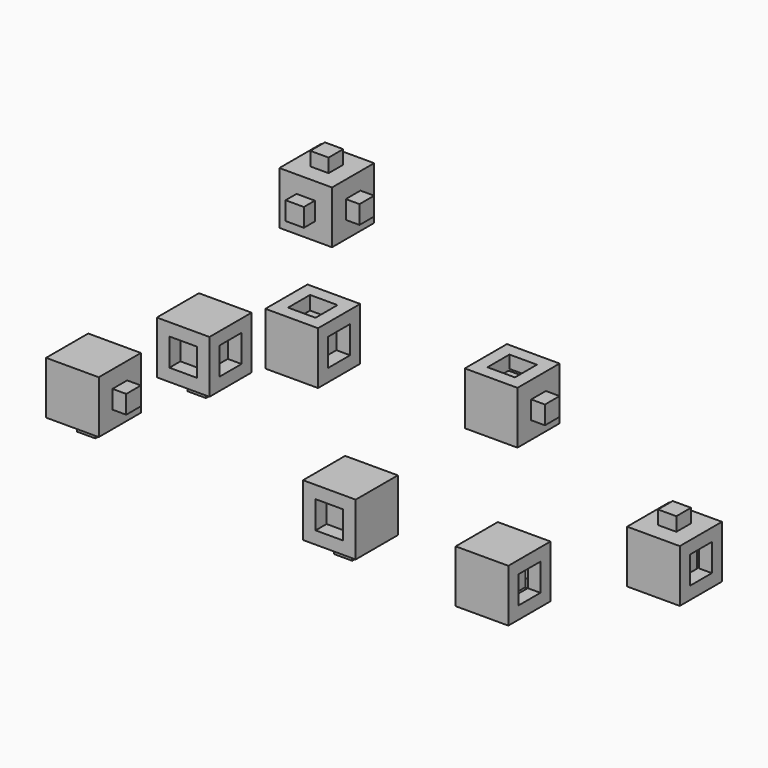
from build123d import *

# Parameters (mm, degrees)
F0_W      = 5.75
F0_H      = 5.75
F1_DEPTH  = 5.75
F2_W      = 3
F2_H      = 3
F4_DEPTH  = 1.5
F3_W      = 2
F3_H      = 2
F5_DEPTH  = 1.5
F6_W      = 3
F6_H      = 3
F7_DEPTH  = 1.5
F8_W      = 2
F8_H      = 2
F9_DEPTH  = 1.5
F10_W     = 2
F10_H     = 2
F11_DEPTH = 1.5
F12_W     = 2
F12_H     = 2
F13_DEPTH = 1.5
F14_W     = 3
F14_H     = 3
F15_DEPTH = 1.5
F16_W     = 2
F16_H     = 2
F17_DEPTH = 1.5
F18_W     = 2
F18_H     = 2
F19_DEPTH = 1.5
F20_W     = 3
F20_H     = 3
F21_DEPTH = 1.5
F22_W     = 3
F22_H     = 3
F23_DEPTH = 1.5
F24_DEPTH = 1.5
F25_W     = 2
F25_H     = 2
F26_DEPTH = 1.5
F28_W     = 2
F28_H     = 2
F29_DEPTH = 1.5
F27_W     = 2
F27_H     = 2
F30_DEPTH = 1.5
F31_W     = 2
F31_H     = 2
F32_DEPTH = 1.5
F33_W     = 3
F33_H     = 3
F34_DEPTH = 1.5
F35_W     = 3
F35_H     = 3
F36_DEPTH = 1.5
F37_W     = 2
F37_H     = 2
F38_DEPTH = 1.5
F39_W     = 2
F39_H     = 2
F40_DEPTH = 1.5
F41_W     = 3
F41_H     = 3
F42_DEPTH = 1.5
F43_W     = 3
F43_H     = 3
F44_DEPTH = 1.5
F45_W     = 3
F45_H     = 3
F46_DEPTH = 1.5
F47_W     = 3
F47_H     = 3
F48_DEPTH = 1.5
F49_W     = 3
F49_H     = 3
F50_DEPTH = 1.5


# Not quite as in the source:
# - a feature names something its author has since deleted; it is built from what else it names


with BuildPart() as f1:
    # F0 (on Front) → F1 (new body)
    with BuildSketch(Plane.XZ):
        with Locations((-12.646038468, 21.76645218)):
            Rectangle(F0_W, F0_H)
    extrude(amount=F1_DEPTH)

    # F22 (on face) → F24 (cut)
    with BuildSketch(Plane(origin=(0, 0, 0), x_dir=(-1, 0, 0), z_dir=(0, 1, 0))):
        with Locations((-25.3156977051, -0.3534462649)):
            Rectangle(F22_W, F22_H)
    extrude(amount=-F24_DEPTH, mode=Mode.SUBTRACT)

    # F28 (on face) → F29 (join)
    with BuildSketch(Plane.XY.offset(24.64145218)):
        with Locations((-12.646038468, -2.875)):
            Rectangle(F28_W, F28_H)
    extrude(amount=F29_DEPTH)

    # F27 (on face) → F30 (join)
    with BuildSketch(Plane.XZ.offset(5.75)):
        with Locations((-12.646038468, 21.76645218)):
            Rectangle(F27_W, F27_H)
    extrude(amount=F30_DEPTH)

    # F31 (on face) → F32 (join)
    with BuildSketch(Plane.YZ.offset(-9.771038468)):
        with Locations((-2.875, 21.76645218)):
            Rectangle(F31_W, F31_H)
    extrude(amount=F32_DEPTH)


with BuildPart() as f1b:
    # F0 (on Front) → F1, piece 2 (new body)
    with BuildSketch(Plane.XZ):
        with Locations((-14.1715484071, 7.7434927479)):
            Rectangle(F0_W, F0_H)
    extrude(amount=F1_DEPTH)

    # F39 (on face) → F40 (join)
    with BuildSketch(Plane(origin=(0, 0, 0), x_dir=(-1, 0, 0), z_dir=(0, 1, 0))):
        with Locations((14.1715484071, 7.7434927479)):
            Rectangle(F39_W, F39_H)
    extrude(amount=F40_DEPTH)

    # F41 (on face) → F42 (cut)
    with BuildSketch(Plane.XY.offset(10.6184927479)):
        with Locations((-14.1715484071, -2.875)):
            Rectangle(F41_W, F41_H)
    extrude(amount=-F42_DEPTH, mode=Mode.SUBTRACT)

    # F43 (on face) → F44 (cut)
    with BuildSketch(Plane.YZ.offset(-11.2965484071)):
        with Locations((-2.875, 7.7434927479)):
            Rectangle(F43_W, F43_H)
    extrude(amount=-F44_DEPTH, mode=Mode.SUBTRACT)


with BuildPart() as f1c:
    # F0 (on Front) → F1, piece 3 (new body)
    with BuildSketch(Plane.XZ):
        with Locations((-26.0235892455, 3.0496152631)):
            Rectangle(F0_W, F0_H)
    extrude(amount=F1_DEPTH)

    # F2 (on face) → F4 (cut)
    with BuildSketch(Plane.XZ.offset(5.75)):
        with Locations((-26.0235892455, 3.0496152631)):
            Rectangle(F2_W, F2_H)
    extrude(amount=-F4_DEPTH, mode=Mode.SUBTRACT)

    # F3 (on face) → F5 (join)
    with BuildSketch(Plane(origin=(0, 0, 0.1746152631), x_dir=(1, 0, 0), z_dir=(0, 0, -1))):
        with Locations((-26.0235892455, 2.875)):
            Rectangle(F3_W, F3_H)
    extrude(amount=F5_DEPTH)

    # F6 (on face) → F7 (cut)
    with BuildSketch(Plane.YZ.offset(-23.1485892455)):
        with Locations((-2.875, 3.0496152631)):
            Rectangle(F6_W, F6_H)
    extrude(amount=-F7_DEPTH, mode=Mode.SUBTRACT)


with BuildPart() as f1d:
    # F0 (on Front) → F1, piece 4 (new body)
    with BuildSketch(Plane.XZ):
        with Locations((-38.1103243368, -4.7539562041)):
            Rectangle(F0_W, F0_H)
    extrude(amount=F1_DEPTH)

    # F8 (on face) → F9 (join)
    with BuildSketch(Plane(origin=(0, 0, 0), x_dir=(-1, 0, 0), z_dir=(0, 1, 0))):
        with Locations((38.1103243368, -4.7539562041)):
            Rectangle(F8_W, F8_H)
    extrude(amount=F9_DEPTH)

    # F10 (on face) → F11 (join)
    with BuildSketch(Plane.YZ.offset(-35.2353243368)):
        with Locations((-2.875, -4.7539562041)):
            Rectangle(F10_W, F10_H)
    extrude(amount=F11_DEPTH)

    # F12 (on face) → F13 (join)
    with BuildSketch(Plane(origin=(0, 0, -7.6289562041), x_dir=(1, 0, 0), z_dir=(0, 0, -1))):
        with Locations((-38.1103243368, 2.875)):
            Rectangle(F12_W, F12_H)
    extrude(amount=F13_DEPTH)


with BuildPart() as f1e:
    # F0 (on Front) → F1, piece 5 (new body)
    with BuildSketch(Plane.XZ):
        with Locations((-10.0644060136, -7.3942619512)):
            Rectangle(F0_W, F0_H)
    extrude(amount=F1_DEPTH)

    # F14 (on face) → F15 (cut)
    with BuildSketch(Plane.XZ.offset(5.75)):
        with Locations((-10.0644060136, -7.3942619512)):
            Rectangle(F14_W, F14_H)
    extrude(amount=-F15_DEPTH, mode=Mode.SUBTRACT)

    # F16 (on face) → F17 (join)
    with BuildSketch(Plane(origin=(0, 0, -10.2692619512), x_dir=(1, 0, 0), z_dir=(0, 0, -1))):
        with Locations((-10.0644060136, 2.875)):
            Rectangle(F16_W, F16_H)
    extrude(amount=F17_DEPTH)

    # F18 (on face) → F19 (join)
    with BuildSketch(Plane(origin=(-12.9394060136, 0, 0), x_dir=(0, -1, 0), z_dir=(-1, 0, 0))):
        with Locations((2.875, -7.3942619512)):
            Rectangle(F18_W, F18_H)
    extrude(amount=F19_DEPTH)


with BuildPart() as f1f:
    # F0 (on Front) → F1, piece 6 (new body)
    with BuildSketch(Plane.XZ):
        with Locations((6.5988599769, -8.3330389627)):
            Rectangle(F0_W, F0_H)
    extrude(amount=F1_DEPTH)

    # F45 (on face) → F46 (cut)
    with BuildSketch(Plane.YZ.offset(9.4738599769)):
        with Locations((-2.875, -8.3330389627)):
            Rectangle(F45_W, F45_H)
    extrude(amount=-F46_DEPTH, mode=Mode.SUBTRACT)

    # F47 (on face) → F48 (cut)
    with BuildSketch(Plane(origin=(0, 0, 0), x_dir=(-1, 0, 0), z_dir=(0, 1, 0))):
        with Locations((-6.5988599769, -8.3330389627)):
            Rectangle(F47_W, F47_H)
    extrude(amount=-F48_DEPTH, mode=Mode.SUBTRACT)

    # F49 (on face) → F50 (cut)
    with BuildSketch(Plane(origin=(0, 0, -11.2080389627), x_dir=(1, 0, 0), z_dir=(0, 0, -1))):
        with Locations((6.5988599769, 2.875)):
            Rectangle(F49_W, F49_H)
    extrude(amount=-F50_DEPTH, mode=Mode.SUBTRACT)


with BuildPart() as f1g:
    # F0 (on Front) → F1, piece 7 (new body)
    with BuildSketch(Plane.XZ):
        with Locations((7.5963086585, 9.0929825383)):
            Rectangle(F0_W, F0_H)
    extrude(amount=F1_DEPTH)

    # F33 (on face) → F34 (cut)
    with BuildSketch(Plane.XY.offset(11.9679825383)):
        with Locations((7.5963086585, -2.875)):
            Rectangle(F33_W, F33_H)
    extrude(amount=-F34_DEPTH, mode=Mode.SUBTRACT)

    # F35 (on face) → F36 (cut)
    with BuildSketch(Plane(origin=(0, 0, 0), x_dir=(-1, 0, 0), z_dir=(0, 1, 0))):
        with Locations((-7.5963086585, 9.0929825383)):
            Rectangle(F35_W, F35_H)
    extrude(amount=-F36_DEPTH, mode=Mode.SUBTRACT)

    # F37 (on face) → F38 (join)
    with BuildSketch(Plane.YZ.offset(10.4713086585)):
        with Locations((-2.875, 9.0929825383)):
            Rectangle(F37_W, F37_H)
    extrude(amount=F38_DEPTH)


with BuildPart() as f1h:
    # F0 (on Front) → F1, piece 8 (new body)
    with BuildSketch(Plane.XZ):
        with Locations((25.3156977051, -0.3534462649)):
            Rectangle(F0_W, F0_H)
    extrude(amount=F1_DEPTH)

    # F20 (on face) → F21 (cut)
    with BuildSketch(Plane.YZ.offset(28.1906977051)):
        with Locations((-2.875, -0.3534462649)):
            Rectangle(F20_W, F20_H)
    extrude(amount=-F21_DEPTH, mode=Mode.SUBTRACT)

    # F22 (on face) → F23 (cut)
    with BuildSketch(Plane(origin=(0, 0, 0), x_dir=(-1, 0, 0), z_dir=(0, 1, 0))):
        with Locations((-25.3156977051, -0.3534462649)):
            Rectangle(F22_W, F22_H)
    extrude(amount=-F23_DEPTH, mode=Mode.SUBTRACT)

    # F25 (on face) → F26 (join)
    with BuildSketch(Plane.XY.offset(2.5215537351)):
        with Locations((25.3156977051, -2.875)):
            Rectangle(F25_W, F25_H)
    extrude(amount=F26_DEPTH)


solid = Compound([f1.part, f1b.part, f1c.part, f1d.part, f1e.part, f1f.part, f1g.part, f1h.part])
